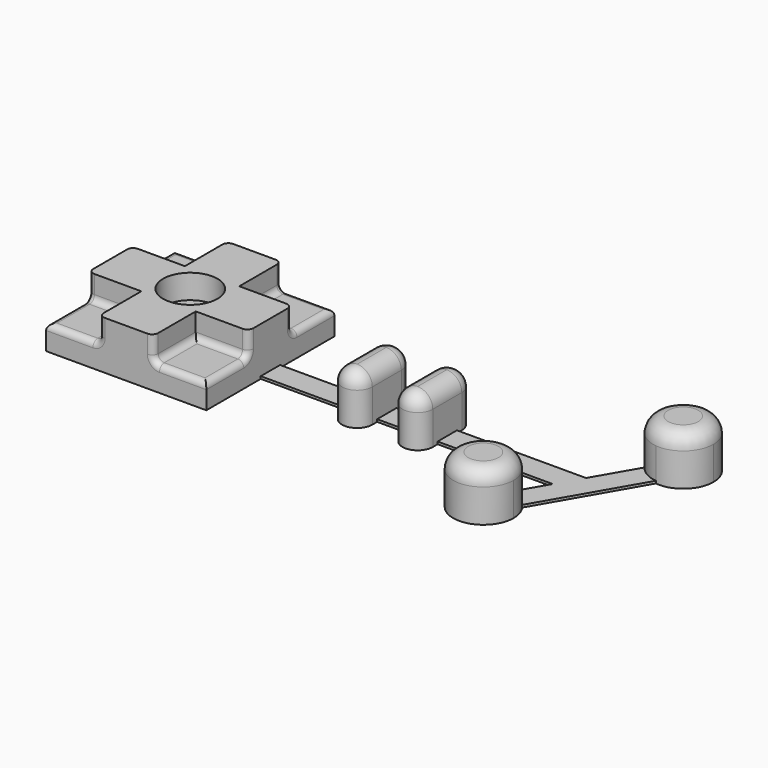
from build123d import *

# Parameters (mm, degrees)
F1_DEPTH     = 8
F0_W         = 14.25
F0_H         = 4
F0_W_2       = 5
F2_DEPTH     = 0.4
F3_T1_DEPTH  = 6
F3_T8_ANGLE  = 180
F3_T10_ANGLE = 180
F3_T12_ANGLE = 180
F3_T14_ANGLE = 180
F4_R         = 4.5
F4_W         = 8.75
F4_H         = 8.75
F5_DEPTH     = 4
F6_F1_R      = 1
F6_F2_R      = 1


# Not quite as in the source:
# - a fillet or chamfer that OpenCascade refuses, or shapes differently, is made with other operations: its cross-section is extruded or revolved along the edge and cut away or added


with BuildPart() as f1:
    # F0 (on Top) → F1 (new body)
    with BuildSketch(Plane.XY):
        Polygon((13.25, 2), (13.25, 13.25), (-13.25, 13.25), (-13.25, -13.25), (13.25, -13.25), (13.25, -2), align=None)
    extrude(amount=F1_DEPTH)



with BuildPart() as f1b:
    # F0 (on Top) → F1, piece 2 (new body)
    with BuildSketch(Plane.XY):
        with BuildLine():
            ThreePointArc((76.9282032303, 12), (70.3656241563, 16.7495627838), (67.9048645752, 9.0313730334))
            ThreePointArc((67.9048645752, 9.0313730334), (69.4282032303, 7.6698729811), (71.3689661904, 7.0313730334))
            ThreePointArc((71.3689661904, 7.0313730334), (75.260155721, 8.2719854346), (76.9282032303, 12))
        make_face()
    extrude(amount=F1_DEPTH)


with BuildPart() as f1c:
    # F0 (on Top) → F1, piece 3 (new body)
    with BuildSketch(Plane.XY):
        with BuildLine():
            ThreePointArc((62.0951354248, -9.0313730334), (60.5717967697, -7.6698729811), (58.6310338096, -7.0313730334))
            ThreePointArc((58.6310338096, -7.0313730334), (54.3437822043, -15.3319524907), (63.0717967697, -12))
            ThreePointArc((63.0717967697, -12), (62.8213595536, -10.437420926), (62.0951354248, -9.0313730334))
        make_face()
    extrude(amount=F1_DEPTH)


with BuildPart() as f1d:
    # F0 (on Top) → F1, piece 4 (new body)
    with BuildSketch(Plane.XY):
        with BuildLine():
            Line((27.5, 3), (27.5, 2))
            Line((27.5, 2), (27.5, -2))
            Line((27.5, -2), (27.5, -3))
            ThreePointArc((27.5, -3), (30, -5.5), (32.5, -3))
            Line((32.5, -3), (32.5, -2))
            Line((32.5, -2), (32.5, 2))
            Line((32.5, 2), (32.5, 3))
            ThreePointArc((32.5, 3), (30, 5.5), (27.5, 3))
        make_face()
    extrude(amount=F1_DEPTH)


with BuildPart() as f1e:
    # F0 (on Top) → F1, piece 5 (new body)
    with BuildSketch(Plane.XY):
        with BuildLine():
            Line((37.5, 3), (37.5, 2))
            Line((37.5, 2), (37.5, -2))
            Line((37.5, -2), (37.5, -3))
            ThreePointArc((37.5, -3), (40, -5.5), (42.5, -3))
            Line((42.5, -3), (42.5, -2))
            Line((42.5, -2), (42.5, 2))
            Line((42.5, 2), (42.5, 3))
            ThreePointArc((42.5, 3), (40, 5.5), (37.5, 3))
        make_face()
    extrude(amount=F1_DEPTH)


with BuildPart() as f1_1:
    add(f1.part)

    add(f1b.part)  # F2 merges F1b

    add(f1c.part)  # F2 merges F1c

    add(f1d.part)  # F2 merges F1d

    add(f1e.part)  # F2 merges F1e
    # F0 (on Top) → F2 (join)
    with BuildSketch(Plane.XY):
        with Locations((20.375, 0)):
            Rectangle(F0_W, F0_H)
        with Locations((35, 0)):
            Rectangle(F0_W_2, F0_H)
        Polygon((63.8452994616, 2), (42.5, 2), (42.5, -2), (61.5358983849, -2), align=None)
        with BuildLine():
            Line((67.9048645752, 9.0313730334), (63.8452994616, 2))
            Line((63.8452994616, 2), (61.5358983849, -2))
            Line((61.5358983849, -2), (58.6310338096, -7.0313730334))
            ThreePointArc((58.6310338096, -7.0313730334), (60.5717967697, -7.6698729811), (62.0951354248, -9.0313730334))
            Line((62.0951354248, -9.0313730334), (71.3689661904, 7.0313730334))
            ThreePointArc((71.3689661904, 7.0313730334), (69.4282032303, 7.6698729811), (67.9048645752, 9.0313730334))
        make_face()
    extrude(amount=F2_DEPTH)

    # F3: fillet of radius 2.5 on 10 edges, made by hand

    # F3_s2 → F3_t1 (cut)
    with BuildSketch(Plane.XZ.offset(-3)):
        with BuildLine():
            ThreePointArc((37.5, 5.5), (38.232233047, 7.267766953), (40, 8))
            Line((40, 8), (37.5, 8))
            Line((37.5, 8), (37.5, 5.5))
        make_face()
        with BuildLine():
            ThreePointArc((42.5, 5.5), (41.767766953, 7.267766953), (40, 8))
            Line((40, 8), (42.5, 8))
            Line((42.5, 8), (42.5, 5.5))
        make_face()
        with BuildLine():
            ThreePointArc((27.5, 5.5), (28.232233047, 7.267766953), (30, 8))
            Line((30, 8), (27.5, 8))
            Line((27.5, 8), (27.5, 5.5))
        make_face()
        with BuildLine():
            ThreePointArc((32.5, 5.5), (31.767766953, 7.267766953), (30, 8))
            Line((30, 8), (32.5, 8))
            Line((32.5, 8), (32.5, 5.5))
        make_face()
    extrude(amount=F3_T1_DEPTH, mode=Mode.SUBTRACT)

    # F3_s3 → F3_t4 (revolve, cut)
    with BuildSketch(Plane.XZ.offset(12)):
        with BuildLine():
            ThreePointArc((63.0717967697, 5.5), (62.3395637227, 7.267766953), (60.5717967697, 8))
            Line((60.5717967697, 8), (63.0717967697, 8))
            Line((63.0717967697, 8), (63.0717967697, 5.5))
        make_face()
    revolve(axis=Axis((58.0717967697, -12, 8), (0, 0, -1)), mode=Mode.SUBTRACT)

    # F3_s5 → F3_t6 (revolve, cut)
    with BuildSketch(Plane(origin=(19.6223796234, -26.5939369719, 0), x_dir=(0, 0, 1), z_dir=(0.5937253933, -0.804667731, 0))):
        with BuildLine():
            ThreePointArc((5.5, -60.0030088087), (7.267766953, -60.7352418558), (8, -62.5030088087))
            Line((8, -62.5030088087), (8, -60.0030088087))
            Line((8, -60.0030088087), (5.5, -60.0030088087))
        make_face()
    revolve(axis=Axis((71.9282032303, 12, 8), (0, 0, -1)), mode=Mode.SUBTRACT)

    # F3_s7 → F3_t8 (revolve, cut)
    with BuildSketch(Plane.XZ.offset(-3)):
        with BuildLine():
            ThreePointArc((42.5, 5.5), (41.767766953, 7.267766953), (40, 8))
            Line((40, 8), (42.5, 8))
            Line((42.5, 8), (42.5, 5.5))
        make_face()
    revolve(axis=Axis((40, 3, 8), (0, 0, 1)), revolution_arc=F3_T8_ANGLE, mode=Mode.SUBTRACT)

    # F3_s9 → F3_t10 (revolve, cut)
    with BuildSketch(Plane.XZ.offset(3)):
        with BuildLine():
            ThreePointArc((40, 8), (38.232233047, 7.267766953), (37.5, 5.5))
            Line((37.5, 5.5), (37.5, 8))
            Line((37.5, 8), (40, 8))
        make_face()
    revolve(axis=Axis((40, -3, 8), (0, 0, 1)), revolution_arc=F3_T10_ANGLE, mode=Mode.SUBTRACT)

    # F3_s11 → F3_t12 (revolve, cut)
    with BuildSketch(Plane.XZ.offset(-3)):
        with BuildLine():
            ThreePointArc((32.5, 5.5), (31.767766953, 7.267766953), (30, 8))
            Line((30, 8), (32.5, 8))
            Line((32.5, 8), (32.5, 5.5))
        make_face()
    revolve(axis=Axis((30, 3, 8), (0, 0, 1)), revolution_arc=F3_T12_ANGLE, mode=Mode.SUBTRACT)

    # F3_s13 → F3_t14 (revolve, cut)
    with BuildSketch(Plane.XZ.offset(3)):
        with BuildLine():
            ThreePointArc((27.5, 5.5), (28.232233047, 7.267766953), (30, 8))
            Line((30, 8), (27.5, 8))
            Line((27.5, 8), (27.5, 5.5))
        make_face()
    revolve(axis=Axis((30, -3, 8), (0, 0, 1)), revolution_arc=F3_T14_ANGLE, mode=Mode.SUBTRACT)

    # F4 (on face) → F5 (cut)
    with BuildSketch(Plane.XY.offset(8)):
        Circle(F4_R)
        with Locations((-8.875, 8.875)):
            Rectangle(F4_W, F4_H)
        with Locations((-8.875, -8.875)):
            Rectangle(F4_W, F4_H)
        with Locations((8.875, -8.875)):
            Rectangle(F4_W, F4_H)
        with Locations((8.875, 8.875)):
            Rectangle(F4_W, F4_H)
    extrude(amount=-F5_DEPTH, mode=Mode.SUBTRACT)

    # F6: fillet of radius 1 on 16 edges, made by hand

    # F6_f1
    f6_f1_edges = [f1_1.edges().sort_by_distance(p)[0] for p in [
        (8.875, -4.5, 4),
        (4.5, -8.875, 4),
        (4.5, 8.875, 4),
        (8.875, 4.5, 4),
        (-4.5, 8.875, 4),
        (-8.875, 4.5, 4),
        (-8.875, -4.5, 4),
        (-4.5, -8.875, 4),
    ]]
    fillet(f6_f1_edges, radius=F6_F1_R)

    # F6_f2
    f6_f2_edges = [f1_1.edges().sort_by_distance(p)[0] for p in [
        (13.25, -9.375, 4),
        (9.375, -13.25, 4),
        (9.375, 13.25, 4),
        (13.25, 9.375, 4),
        (-9.375, 13.25, 4),
        (-13.25, 9.375, 4),
        (-13.25, -9.375, 4),
        (-9.375, -13.25, 4),
        (-4.7928932188, -13.25, 4.2928932188),
        (-13.25, -4.7928932188, 4.2928932188),
        (-13.25, 4.7928932188, 4.2928932188),
        (-4.7928932188, 13.25, 4.2928932188),
        (13.25, 4.7928932188, 4.2928932188),
        (4.7928932188, 13.25, 4.2928932188),
        (4.7928932188, -13.25, 4.2928932188),
        (13.25, -4.7928932188, 4.2928932188),
    ]]
    fillet(f6_f2_edges, radius=F6_F2_R)


solid = f1_1.part
